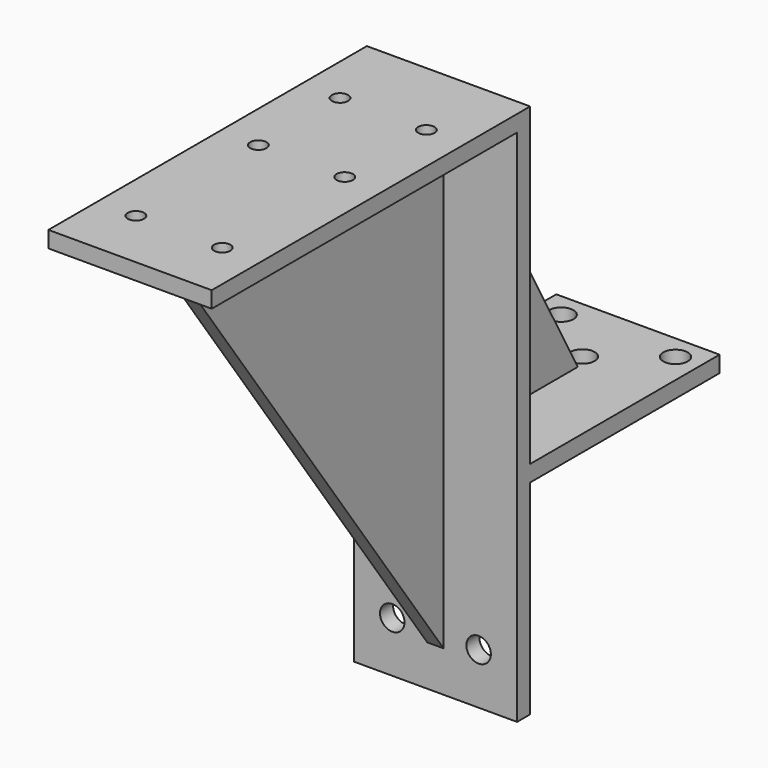
from build123d import *

# Parameters (mm, degrees)
F1_DEPTH = 40
F2_DEPTH = 4
F3_R     = 4
F4_DEPTH = 262.201
F5_R     = 6
F6_DEPTH = 124.001
F7_R     = 6
F8_DEPTH = 108.001


# Not quite as in the source:
# - a pattern or mirror of a feature is missing from the dataset's text; its kind, count and spacing are read off the source's solid


with BuildPart() as f1:
    # F0 (on Right) → F1 (new body, symmetric)
    with BuildSketch(Plane.YZ):
        Polygon((0, 262.2), (-195, 262.2), (-195, 254.2), (-175, 254.2), (-8, 254.2), (-8, 20), (-8, 0), (0, 0), (0, 100), (0, 108), (0, 242.2), align=None)
        Polygon((74.1, 108), (0, 108), (0, 100), (116, 100), (116, 108), align=None)
    extrude(amount=F1_DEPTH, both=True)

    # F0 (on Right) → F2 (join, symmetric)
    with BuildSketch(Plane.YZ):
        Polygon((-8, 254.2), (-175, 254.2), (-8, 20), align=None)
        Polygon((74.1, 108), (0, 242.2), (0, 108), align=None)
    extrude(amount=F2_DEPTH, both=True)

    # F3 (on face) → F4 (cut, through all)
    with BuildSketch(Plane.XY.offset(262.2)):
        with Locations((-21.15, -40)):
            Circle(F3_R)
        with Locations((-21.15, -90)):
            Circle(F3_R)
        with Locations((-21.15, -165)):
            Circle(F3_R)
    f4 = extrude(amount=-F4_DEPTH, mode=Mode.SUBTRACT)

    # F4_copies: F4 across plane
    add(f4.mirror(Plane(origin=(0, 0, 0), x_dir=(0, 0, 1), z_dir=(1, 0, 0))), mode=Mode.SUBTRACT)

    # F5 (on face) → F6 (cut, through all)
    with BuildSketch(Plane.XZ.offset(8)):
        with Locations((-21.15, 25)):
            Circle(F5_R)
    f6 = extrude(amount=-F6_DEPTH, mode=Mode.SUBTRACT)

    # F6_copies: F6 across plane
    add(f6.mirror(Plane(origin=(0, 0, 0), x_dir=(0, 0, 1), z_dir=(1, 0, 0))), mode=Mode.SUBTRACT)

    # F7 (on face) → F8 (cut, through all)
    with BuildSketch(Plane.XY.offset(108)):
        with Locations((-28, 104)):
            Circle(F7_R)
        with Locations((0, 82)):
            Circle(F7_R)
        with Locations((28, 104)):
            Circle(F7_R)
    extrude(amount=-F8_DEPTH, mode=Mode.SUBTRACT)


solid = f1.part
